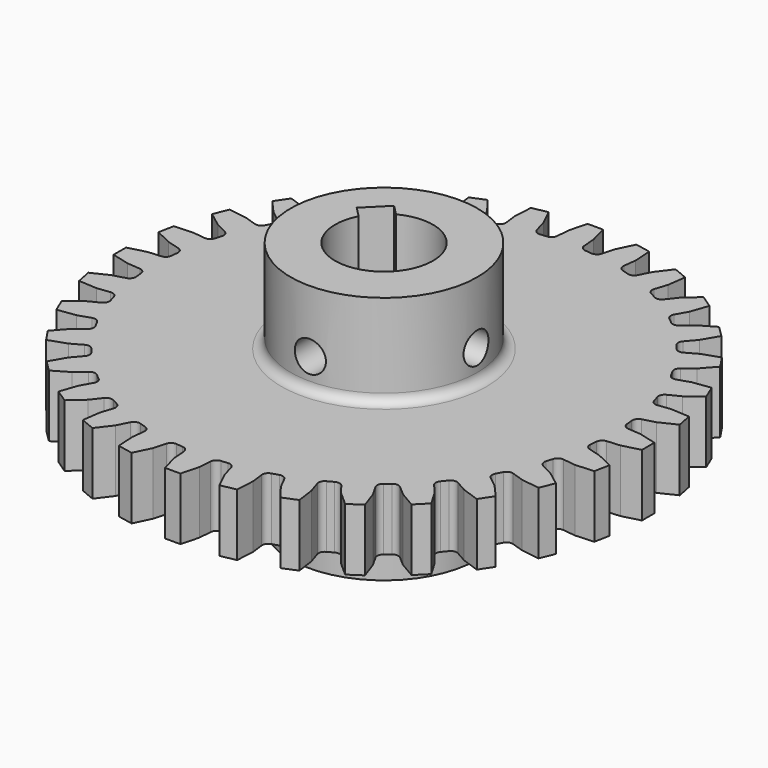
from build123d import *

# Parameters (mm, degrees)
F1_DEPTH      = 12.7
F2_R          = 1.27
F3_R          = 19.05
F4_DEPTH      = 19.05
F4_DEPTH_BACK = 31.75
F5_DEPTH      = 25.4
F6_R          = 1.905
F7_R          = 3.175
F8_DEPTH      = 25.4
F9_R          = 3.175
F10_DEPTH     = 25.4


with BuildPart() as f1:
    # F0 (on Top) → F1 (new body)
    with BuildSketch(Plane.XY):
        with BuildLine():
            Line((-2.54, 50.3120746804), (-2.8220822748, 46.587102377))
            ThreePointArc((-2.8220822748, 46.587102377), (-4.574704982, 46.4477591556), (-6.3208360493, 46.2425052077))
            Line((-6.3208360493, 46.2425052077), (-7.3242042385, 49.840871691))
            Line((-7.3242042385, 49.840871691), (-8.9684480145, 53.2246894327))
            Line((-8.9684480145, 53.2246894327), (-12.0824412797, 52.6052776603))
            Line((-12.0824412797, 52.6052776603), (-12.3065934629, 48.8498128552))
            Line((-12.3065934629, 48.8498128552), (-11.8565495597, 45.1413833282))
            ThreePointArc((-11.8565495597, 45.1413833282), (-13.5483115992, 44.6627978195), (-15.2208481888, 44.1208344964))
            Line((-15.2208481888, 44.1208344964), (-16.9069434155, 47.4543119536))
            Line((-16.9069434155, 47.4543119536), (-19.1797436013, 50.4523345385))
            Line((-19.1797436013, 50.4523345385), (-22.113061117, 49.2373146408))
            Line((-22.113061117, 49.2373146408), (-21.6002514407, 45.5102801172))
            Line((-21.6002514407, 45.5102801172), (-20.4353762943, 41.9609062338))
            ThreePointArc((-20.4353762943, 41.9609062338), (-22.0012641995, 41.1614702103), (-23.5359316684, 40.3036248587))
            Line((-23.5359316684, 40.3036248587), (-25.8399582386, 43.2441096205))
            Line((-25.8399582386, 43.2441096205), (-28.6539723976, 45.741124722))
            Line((-28.6539723976, 45.741124722), (-31.2938884167, 43.9771892322))
            Line((-31.2938884167, 43.9771892322), (-30.0638238691, 40.4218128368))
            Line((-30.0638238691, 40.4218128368), (-28.2288829782, 37.1678950447))
            ThreePointArc((-28.2288829782, 37.1678950447), (-29.6087205551, 36.0783303846), (-30.946542493, 34.9375695202))
            Line((-30.946542493, 34.9375695202), (-33.7799579579, 37.3720604063))
            Line((-33.7799579579, 37.3720604063), (-37.0270451041, 39.2721091343))
            Line((-37.0270451041, 39.2721091343), (-39.2721091343, 37.0270451041))
            Line((-39.2721091343, 37.0270451041), (-37.3720604063, 33.7799579579))
            Line((-37.3720604063, 33.7799579579), (-34.9375695202, 30.946542493))
            ThreePointArc((-34.9375695202, 30.946542493), (-36.0783303846, 29.6087205551), (-37.1678950447, 28.2288829782))
            Line((-37.1678950447, 28.2288829782), (-40.4218128368, 30.0638238691))
            Line((-40.4218128368, 30.0638238691), (-43.9771892322, 31.2938884167))
            Line((-43.9771892322, 31.2938884167), (-45.741124722, 28.6539723976))
            Line((-45.741124722, 28.6539723976), (-43.2441096205, 25.8399582386))
            Line((-43.2441096205, 25.8399582386), (-40.3036248587, 23.5359316684))
            ThreePointArc((-40.3036248587, 23.5359316684), (-41.1614702103, 22.0012641995), (-41.9609062338, 20.4353762943))
            Line((-41.9609062338, 20.4353762943), (-45.5102801172, 21.6002514407))
            Line((-45.5102801172, 21.6002514407), (-49.2373146408, 22.113061117))
            Line((-49.2373146408, 22.113061117), (-50.4523345385, 19.1797436013))
            Line((-50.4523345385, 19.1797436013), (-47.4543119536, 16.9069434155))
            Line((-47.4543119536, 16.9069434155), (-44.1208344964, 15.2208481888))
            ThreePointArc((-44.1208344964, 15.2208481888), (-44.6627978195, 13.5483115992), (-45.1413833282, 11.8565495597))
            Line((-45.1413833282, 11.8565495597), (-48.8498128552, 12.3065934629))
            Line((-48.8498128552, 12.3065934629), (-52.6052776603, 12.0824412797))
            Line((-52.6052776603, 12.0824412797), (-53.2246894327, 8.9684480145))
            Line((-53.2246894327, 8.9684480145), (-49.840871691, 7.3242042385))
            Line((-49.840871691, 7.3242042385), (-46.2425052077, 6.3208360493))
            ThreePointArc((-46.2425052077, 6.3208360493), (-46.4477591556, 4.574704982), (-46.587102377, 2.8220822748))
            Line((-46.587102377, 2.8220822748), (-50.3120746804, 2.54))
            Line((-50.3120746804, 2.54), (-53.9516493608, 1.5875))
            Line((-53.9516493608, 1.5875), (-53.9516493608, -1.5875))
            Line((-53.9516493608, -1.5875), (-50.3120746804, -2.54))
            Line((-50.3120746804, -2.54), (-46.587102377, -2.8220822748))
            ThreePointArc((-46.587102377, -2.8220822748), (-46.4477591556, -4.574704982), (-46.2425052077, -6.3208360493))
            Line((-46.2425052077, -6.3208360493), (-49.840871691, -7.3242042385))
            Line((-49.840871691, -7.3242042385), (-53.2246894327, -8.9684480145))
            Line((-53.2246894327, -8.9684480145), (-52.6052776603, -12.0824412797))
            Line((-52.6052776603, -12.0824412797), (-48.8498128552, -12.3065934629))
            Line((-48.8498128552, -12.3065934629), (-45.1413833282, -11.8565495597))
            ThreePointArc((-45.1413833282, -11.8565495597), (-44.6627978195, -13.5483115992), (-44.1208344964, -15.2208481888))
            Line((-44.1208344964, -15.2208481888), (-47.4543119536, -16.9069434155))
            Line((-47.4543119536, -16.9069434155), (-50.4523345385, -19.1797436013))
            Line((-50.4523345385, -19.1797436013), (-49.2373146408, -22.113061117))
            Line((-49.2373146408, -22.113061117), (-45.5102801172, -21.6002514407))
            Line((-45.5102801172, -21.6002514407), (-41.9609062338, -20.4353762943))
            ThreePointArc((-41.9609062338, -20.4353762943), (-41.1614702103, -22.0012641995), (-40.3036248587, -23.5359316684))
            Line((-40.3036248587, -23.5359316684), (-43.2441096205, -25.8399582386))
            Line((-43.2441096205, -25.8399582386), (-45.741124722, -28.6539723976))
            Line((-45.741124722, -28.6539723976), (-43.9771892322, -31.2938884167))
            Line((-43.9771892322, -31.2938884167), (-40.4218128368, -30.0638238691))
            Line((-40.4218128368, -30.0638238691), (-37.1678950447, -28.2288829782))
            ThreePointArc((-37.1678950447, -28.2288829782), (-36.0783303846, -29.6087205551), (-34.9375695202, -30.946542493))
            Line((-34.9375695202, -30.946542493), (-37.3720604063, -33.7799579579))
            Line((-37.3720604063, -33.7799579579), (-39.2721091343, -37.0270451041))
            Line((-39.2721091343, -37.0270451041), (-37.0270451041, -39.2721091343))
            Line((-37.0270451041, -39.2721091343), (-33.7799579579, -37.3720604063))
            Line((-33.7799579579, -37.3720604063), (-30.946542493, -34.9375695202))
            ThreePointArc((-30.946542493, -34.9375695202), (-29.6087205551, -36.0783303846), (-28.2288829782, -37.1678950447))
            Line((-28.2288829782, -37.1678950447), (-30.0638238691, -40.4218128368))
            Line((-30.0638238691, -40.4218128368), (-31.2938884167, -43.9771892322))
            Line((-31.2938884167, -43.9771892322), (-28.6539723976, -45.741124722))
            Line((-28.6539723976, -45.741124722), (-25.8399582386, -43.2441096205))
            Line((-25.8399582386, -43.2441096205), (-23.5359316684, -40.3036248587))
            ThreePointArc((-23.5359316684, -40.3036248587), (-22.0012641995, -41.1614702103), (-20.4353762943, -41.9609062338))
            Line((-20.4353762943, -41.9609062338), (-21.6002514407, -45.5102801172))
            Line((-21.6002514407, -45.5102801172), (-22.113061117, -49.2373146408))
            Line((-22.113061117, -49.2373146408), (-19.1797436013, -50.4523345385))
            Line((-19.1797436013, -50.4523345385), (-16.9069434155, -47.4543119536))
            Line((-16.9069434155, -47.4543119536), (-15.2208481888, -44.1208344964))
            ThreePointArc((-15.2208481888, -44.1208344964), (-13.5483115992, -44.6627978195), (-11.8565495597, -45.1413833282))
            Line((-11.8565495597, -45.1413833282), (-12.3065934629, -48.8498128552))
            Line((-12.3065934629, -48.8498128552), (-12.0824412797, -52.6052776603))
            Line((-12.0824412797, -52.6052776603), (-8.9684480145, -53.2246894327))
            Line((-8.9684480145, -53.2246894327), (-7.3242042385, -49.840871691))
            Line((-7.3242042385, -49.840871691), (-6.3208360493, -46.2425052077))
            ThreePointArc((-6.3208360493, -46.2425052077), (-4.574704982, -46.4477591556), (-2.8220822748, -46.587102377))
            Line((-2.8220822748, -46.587102377), (-2.54, -50.3120746804))
            Line((-2.54, -50.3120746804), (-1.5875, -53.9516493608))
            Line((-1.5875, -53.9516493608), (1.5875, -53.9516493608))
            Line((1.5875, -53.9516493608), (2.54, -50.3120746804))
            Line((2.54, -50.3120746804), (2.8220822748, -46.587102377))
            ThreePointArc((2.8220822748, -46.587102377), (4.574704982, -46.4477591556), (6.3208360493, -46.2425052077))
            Line((6.3208360493, -46.2425052077), (7.3242042385, -49.840871691))
            Line((7.3242042385, -49.840871691), (8.9684480145, -53.2246894327))
            Line((8.9684480145, -53.2246894327), (12.0824412797, -52.6052776603))
            Line((12.0824412797, -52.6052776603), (12.3065934629, -48.8498128552))
            Line((12.3065934629, -48.8498128552), (11.8565495597, -45.1413833282))
            ThreePointArc((11.8565495597, -45.1413833282), (13.5483115992, -44.6627978195), (15.2208481888, -44.1208344964))
            Line((15.2208481888, -44.1208344964), (16.9069434155, -47.4543119536))
            Line((16.9069434155, -47.4543119536), (19.1797436013, -50.4523345385))
            Line((19.1797436013, -50.4523345385), (22.113061117, -49.2373146408))
            Line((22.113061117, -49.2373146408), (21.6002514407, -45.5102801172))
            Line((21.6002514407, -45.5102801172), (20.4353762943, -41.9609062338))
            ThreePointArc((20.4353762943, -41.9609062338), (22.0012641995, -41.1614702103), (23.5359316684, -40.3036248587))
            Line((23.5359316684, -40.3036248587), (25.8399582386, -43.2441096205))
            Line((25.8399582386, -43.2441096205), (28.6539723976, -45.741124722))
            Line((28.6539723976, -45.741124722), (31.2938884167, -43.9771892322))
            Line((31.2938884167, -43.9771892322), (30.0638238691, -40.4218128368))
            Line((30.0638238691, -40.4218128368), (28.2288829782, -37.1678950447))
            ThreePointArc((28.2288829782, -37.1678950447), (29.6087205551, -36.0783303846), (30.946542493, -34.9375695202))
            Line((30.946542493, -34.9375695202), (33.7799579579, -37.3720604063))
            Line((33.7799579579, -37.3720604063), (37.0270451041, -39.2721091343))
            Line((37.0270451041, -39.2721091343), (39.2721091343, -37.0270451041))
            Line((39.2721091343, -37.0270451041), (37.3720604063, -33.7799579579))
            Line((37.3720604063, -33.7799579579), (34.9375695202, -30.946542493))
            ThreePointArc((34.9375695202, -30.946542493), (36.0783303846, -29.6087205551), (37.1678950447, -28.2288829782))
            Line((37.1678950447, -28.2288829782), (40.4218128368, -30.0638238691))
            Line((40.4218128368, -30.0638238691), (43.9771892322, -31.2938884167))
            Line((43.9771892322, -31.2938884167), (45.741124722, -28.6539723976))
            Line((45.741124722, -28.6539723976), (43.2441096205, -25.8399582386))
            Line((43.2441096205, -25.8399582386), (40.3036248587, -23.5359316684))
            ThreePointArc((40.3036248587, -23.5359316684), (41.1614702103, -22.0012641995), (41.9609062338, -20.4353762943))
            Line((41.9609062338, -20.4353762943), (45.5102801172, -21.6002514407))
            Line((45.5102801172, -21.6002514407), (49.2373146408, -22.113061117))
            Line((49.2373146408, -22.113061117), (50.4523345385, -19.1797436013))
            Line((50.4523345385, -19.1797436013), (47.4543119536, -16.9069434155))
            Line((47.4543119536, -16.9069434155), (44.1208344964, -15.2208481888))
            ThreePointArc((44.1208344964, -15.2208481888), (44.6627978195, -13.5483115992), (45.1413833282, -11.8565495597))
            Line((45.1413833282, -11.8565495597), (48.8498128552, -12.3065934629))
            Line((48.8498128552, -12.3065934629), (52.6052776603, -12.0824412797))
            Line((52.6052776603, -12.0824412797), (53.2246894327, -8.9684480145))
            Line((53.2246894327, -8.9684480145), (49.840871691, -7.3242042385))
            Line((49.840871691, -7.3242042385), (46.2425052077, -6.3208360493))
            ThreePointArc((46.2425052077, -6.3208360493), (46.4477591556, -4.574704982), (46.587102377, -2.8220822748))
            Line((46.587102377, -2.8220822748), (50.3120746804, -2.54))
            Line((50.3120746804, -2.54), (53.9516493608, -1.5875))
            Line((53.9516493608, -1.5875), (53.9516493608, 1.5875))
            Line((53.9516493608, 1.5875), (50.3120746804, 2.54))
            Line((50.3120746804, 2.54), (46.587102377, 2.8220822748))
            ThreePointArc((46.587102377, 2.8220822748), (46.4477591556, 4.574704982), (46.2425052077, 6.3208360493))
            Line((46.2425052077, 6.3208360493), (49.840871691, 7.3242042385))
            Line((49.840871691, 7.3242042385), (53.2246894327, 8.9684480145))
            Line((53.2246894327, 8.9684480145), (52.6052776603, 12.0824412797))
            Line((52.6052776603, 12.0824412797), (48.8498128552, 12.3065934629))
            Line((48.8498128552, 12.3065934629), (45.1413833282, 11.8565495597))
            ThreePointArc((45.1413833282, 11.8565495597), (44.6627978195, 13.5483115992), (44.1208344964, 15.2208481888))
            Line((44.1208344964, 15.2208481888), (47.4543119536, 16.9069434155))
            Line((47.4543119536, 16.9069434155), (50.4523345385, 19.1797436013))
            Line((50.4523345385, 19.1797436013), (49.2373146408, 22.113061117))
            Line((49.2373146408, 22.113061117), (45.5102801172, 21.6002514407))
            Line((45.5102801172, 21.6002514407), (41.9609062338, 20.4353762943))
            ThreePointArc((41.9609062338, 20.4353762943), (41.1614702103, 22.0012641995), (40.3036248587, 23.5359316684))
            Line((40.3036248587, 23.5359316684), (43.2441096205, 25.8399582386))
            Line((43.2441096205, 25.8399582386), (45.741124722, 28.6539723976))
            Line((45.741124722, 28.6539723976), (43.9771892322, 31.2938884167))
            Line((43.9771892322, 31.2938884167), (40.4218128368, 30.0638238691))
            Line((40.4218128368, 30.0638238691), (37.1678950447, 28.2288829782))
            ThreePointArc((37.1678950447, 28.2288829782), (36.0783303846, 29.6087205551), (34.9375695202, 30.946542493))
            Line((34.9375695202, 30.946542493), (37.3720604063, 33.7799579579))
            Line((37.3720604063, 33.7799579579), (39.2721091343, 37.0270451041))
            Line((39.2721091343, 37.0270451041), (37.0270451041, 39.2721091343))
            Line((37.0270451041, 39.2721091343), (33.7799579579, 37.3720604063))
            Line((33.7799579579, 37.3720604063), (30.946542493, 34.9375695202))
            ThreePointArc((30.946542493, 34.9375695202), (29.6087205551, 36.0783303846), (28.2288829782, 37.1678950447))
            Line((28.2288829782, 37.1678950447), (30.0638238691, 40.4218128368))
            Line((30.0638238691, 40.4218128368), (31.2938884167, 43.9771892322))
            Line((31.2938884167, 43.9771892322), (28.6539723976, 45.741124722))
            Line((28.6539723976, 45.741124722), (25.8399582386, 43.2441096205))
            Line((25.8399582386, 43.2441096205), (23.5359316684, 40.3036248587))
            ThreePointArc((23.5359316684, 40.3036248587), (22.0012641995, 41.1614702103), (20.4353762943, 41.9609062338))
            Line((20.4353762943, 41.9609062338), (21.6002514407, 45.5102801172))
            Line((21.6002514407, 45.5102801172), (22.113061117, 49.2373146408))
            Line((22.113061117, 49.2373146408), (19.1797436013, 50.4523345385))
            Line((19.1797436013, 50.4523345385), (16.9069434155, 47.4543119536))
            Line((16.9069434155, 47.4543119536), (15.2208481888, 44.1208344964))
            ThreePointArc((15.2208481888, 44.1208344964), (13.5483115992, 44.6627978195), (11.8565495597, 45.1413833282))
            Line((11.8565495597, 45.1413833282), (12.3065934629, 48.8498128552))
            Line((12.3065934629, 48.8498128552), (12.0824412797, 52.6052776603))
            Line((12.0824412797, 52.6052776603), (8.9684480145, 53.2246894327))
            Line((8.9684480145, 53.2246894327), (7.3242042385, 49.840871691))
            Line((7.3242042385, 49.840871691), (6.3208360493, 46.2425052077))
            ThreePointArc((6.3208360493, 46.2425052077), (4.574704982, 46.4477591556), (2.8220822748, 46.587102377))
            Line((2.8220822748, 46.587102377), (2.54, 50.3120746804))
            Line((2.54, 50.3120746804), (1.5875, 53.9516493608))
            Line((1.5875, 53.9516493608), (-1.5875, 53.9516493608))
            Line((-1.5875, 53.9516493608), (-2.54, 50.3120746804))
        make_face()
    extrude(amount=F1_DEPTH)

    # F2
    f2_edges = [f1.edges().sort_by_distance(p)[0] for p in [
        (2.822082, 46.587102, 6.35),
        (6.320836, 46.242505, 6.35),
        (11.85655, 45.141383, 6.35),
        (15.220848, 44.120834, 6.35),
        (20.435376, 41.960906, 6.35),
        (23.535932, 40.303625, 6.35),
        (28.228883, 37.167895, 6.35),
        (30.946542, 34.93757, 6.35),
        (34.93757, 30.946542, 6.35),
        (37.167895, 28.228883, 6.35),
        (40.303625, 23.535932, 6.35),
        (41.960906, 20.435376, 6.35),
        (44.120834, 15.220848, 6.35),
        (45.141383, 11.85655, 6.35),
        (46.242505, 6.320836, 6.35),
        (46.587102, 2.822082, 6.35),
        (46.587102, -2.822082, 6.35),
        (46.242505, -6.320836, 6.35),
        (45.141383, -11.85655, 6.35),
        (44.120834, -15.220848, 6.35),
        (41.960906, -20.435376, 6.35),
        (40.303625, -23.535932, 6.35),
        (37.167895, -28.228883, 6.35),
        (34.93757, -30.946542, 6.35),
        (30.946542, -34.93757, 6.35),
        (28.228883, -37.167895, 6.35),
        (23.535932, -40.303625, 6.35),
        (20.435376, -41.960906, 6.35),
        (15.220848, -44.120834, 6.35),
        (11.85655, -45.141383, 6.35),
        (6.320836, -46.242505, 6.35),
        (2.822082, -46.587102, 6.35),
        (-2.822082, -46.587102, 6.35),
        (-6.320836, -46.242505, 6.35),
        (-11.85655, -45.141383, 6.35),
        (-15.220848, -44.120834, 6.35),
        (-20.435376, -41.960906, 6.35),
        (-23.535932, -40.303625, 6.35),
        (-28.228883, -37.167895, 6.35),
        (-30.946542, -34.93757, 6.35),
        (-34.93757, -30.946542, 6.35),
        (-37.167895, -28.228883, 6.35),
        (-40.303625, -23.535932, 6.35),
        (-41.960906, -20.435376, 6.35),
        (-44.120834, -15.220848, 6.35),
        (-45.141383, -11.85655, 6.35),
        (-46.242505, -6.320836, 6.35),
        (-46.587102, -2.822082, 6.35),
        (-46.587102, 2.822082, 6.35),
        (-46.242505, 6.320836, 6.35),
        (-45.141383, 11.85655, 6.35),
        (-44.120834, 15.220848, 6.35),
        (-41.960906, 20.435376, 6.35),
        (-40.303625, 23.535932, 6.35),
        (-37.167895, 28.228883, 6.35),
        (-34.93757, 30.946542, 6.35),
        (-30.946542, 34.93757, 6.35),
        (-28.228883, 37.167895, 6.35),
        (-23.535932, 40.303625, 6.35),
        (-20.435376, 41.960906, 6.35),
        (-15.220848, 44.120834, 6.35),
        (-11.85655, 45.141383, 6.35),
        (-6.320836, 46.242505, 6.35),
        (-2.822082, 46.587102, 6.35),
    ]]
    fillet(f2_edges, radius=F2_R)

    # F3 (on face) → F4 (join, two sides)
    with BuildSketch(Plane.XY.offset(12.7)) as f4_sk:
        Circle(F3_R)
        with BuildLine():
            ThreePointArc((-4.6240484381, 8.8666891252), (7.0710678119, -7.0710678119), (-8.8666891252, 4.6240484381))
            Line((-8.8666891252, 4.6240484381), (-10.9601551084, 6.7175144213))
            Line((-10.9601551084, 6.7175144213), (-6.7175144213, 10.9601551084))
            Line((-6.7175144213, 10.9601551084), (-4.6240484381, 8.8666891252))
        make_face(mode=Mode.SUBTRACT)
    extrude(amount=F4_DEPTH)
    extrude(f4_sk.sketch, amount=-F4_DEPTH_BACK)

    # F5 (cut): a face of the model
    f5_faces = [f1.faces().sort_by_distance(p)[0] for p in [
        (-0.3807905469, 0.3807905469, 0),
    ]]
    extrude(f5_faces, amount=-F5_DEPTH, mode=Mode.SUBTRACT)

    # F6
    f6_edges = [f1.edges().sort_by_distance(p)[0] for p in [
        (-19.05, 0, 12.7),
        (-19.05, 0, 0),
    ]]
    fillet(f6_edges, radius=F6_R)

    # F7 (on Front) → F8 (cut)
    with BuildSketch(Plane.XZ):
        with Locations((0, 19.05)):
            Circle(F7_R)
    extrude(amount=F8_DEPTH, mode=Mode.SUBTRACT)

    # F9 (on Right) → F10 (cut)
    with BuildSketch(Plane.YZ):
        with Locations((0, 19.05)):
            Circle(F9_R)
    extrude(amount=F10_DEPTH, mode=Mode.SUBTRACT)


solid = f1.part
